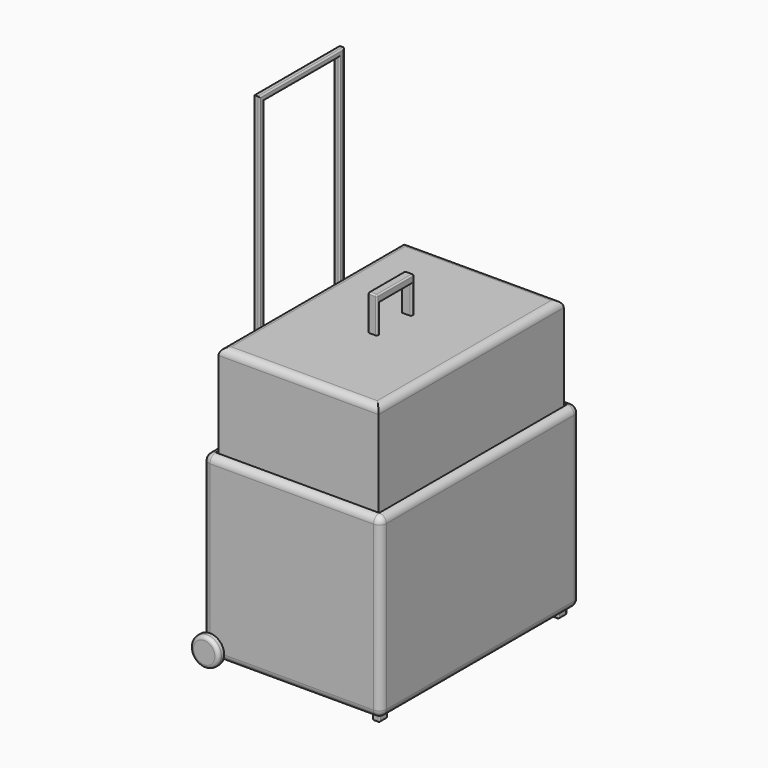
from build123d import *

# Parameters (mm, degrees)
F0_W          = 63.5
F0_H          = 88.9
F1_DEPTH      = 63.5
F2_R          = 2.54
F3_T          = 2.54
F5_W          = 57.1864917874
F5_H          = 82.6394334435
F6_DEPTH      = 63.5
F8_W          = 2.0037387299
F8_H          = 38.1
F9_DEPTH      = 127
F10_W         = 33.6400913075
F10_H         = 121.5383969247
F11_DEPTH     = 25.4
F12_R         = 2.54
F14_R         = 5.08
F15_DEPTH     = 2.54
F17_R         = 5.08
F18_DEPTH     = 2.54
F19_R         = 1.27
F20_R         = 1.27
F21_W         = 2.54
F21_H         = 3.81
F22_DEPTH     = 2.54
F23_T1_DEPTH  = 1.524
F23_T3_DEPTH  = 2.794
F23_T5_DEPTH  = 2.032
F23_S9_W      = 0.51816
F23_S9_H      = 0.51816
F23_T10_DEPTH = 0.51816
F23_S15_W     = 0.51816
F23_S15_H     = 0.51816
F23_T16_DEPTH = 0.51816
F23_S21_W     = 0.51816
F23_S21_H     = 0.51816
F23_T22_DEPTH = 0.51816
F23_S27_W     = 0.51816
F23_S27_H     = 0.51816
F23_T28_DEPTH = 0.51816
F23_T34_DEPTH = 3.302
F23_S35_R     = 2.54
F23_T36_DEPTH = 3
F23_S37_R     = 2.54
F23_T38_DEPTH = 3
F24_W         = 2.54
F24_H         = 3.81
F25_DEPTH     = 2.54
F26_T1_DEPTH  = 2.032
F26_T3_DEPTH  = 1.524
F26_T5_DEPTH  = 2.794
F26_S9_W      = 0.51816
F26_S9_H      = 0.51816
F26_T10_DEPTH = 0.51816
F26_S15_W     = 0.51816
F26_S15_H     = 0.51816
F26_T16_DEPTH = 0.51816
F26_S21_W     = 0.51816
F26_S21_H     = 0.51816
F26_T22_DEPTH = 0.51816
F26_S27_W     = 0.51816
F26_S27_H     = 0.51816
F26_T28_DEPTH = 0.51816
F26_T34_DEPTH = 3.302
F26_S35_R     = 2.54
F26_T36_DEPTH = 3
F26_S37_R     = 2.54
F26_T38_DEPTH = 3
F27_W         = 3.1932555193
F27_H         = 16.5994334435
F28_DEPTH     = 12.7
F29_W         = 14.0208706725
F29_H         = 9.9744812679
F30_DEPTH     = 25.4
F31_R         = 0.508
F32_R         = 0.508
F33_R         = 2.53999
F34_R         = 0.508


# Not quite as in the source:
# - a fillet or chamfer that OpenCascade refuses, or shapes differently, is made with other operations: its cross-section is extruded or revolved along the edge and cut away or added
# - a fillet or chamfer is up to 0.001 mm smaller than in the source, because OpenCascade refuses the exact size
# - a shell that OpenCascade refuses in one call is made with other operations: the cavity is built on its own and cut out


with BuildPart() as f1:
    # F0 (on Top) → F1 (new body)
    with BuildSketch(Plane.XY):
        with Locations((-4.3823961169, -4.1256137789)):
            Rectangle(F0_W, F0_H)
    extrude(amount=F1_DEPTH)

    # F2
    f2_edges = [f1.edges().sort_by_distance(p)[0] for p in [
        (-36.132396, -48.575614, 31.75),
        (27.367604, -48.575614, 31.75),
        (27.367604, 40.324386, 31.75),
        (27.367604, -4.125614, 0),
        (-4.382396, -48.575614, 0),
        (-4.382396, 40.324386, 0),
        (-36.132396, -4.125614, 0),
        (-36.132396, 40.324386, 31.75),
    ]]
    fillet(f2_edges, radius=F2_R)

    # F3: shell of thickness 2.54, made by hand


with BuildPart() as f3_core1:
    # F3_t2: copy of F1
    add(f1.part)

    # the walls: a layer under each face that stays
    f3_faces = [f3_core1.faces().sort_by_distance(p)[0] for p in [
        (-4.3823961169, 40.3243862211, 33.02),
        (27.3676038831, -4.1256137789, 33.02),
        (-36.1323961169, -4.1256137789, 33.02),
        (-4.3823961169, -48.5756137789, 33.02),
        (-4.3823961169, -4.1256137789, 0),
    ]]
    thicken(f3_faces, amount=-F3_T, mode=Mode.SUBTRACT)


with BuildPart() as f1_1:
    add(f1.part)

    # what is left inside the walls is the cavity
    f3_cavity = [f3_core1.part.solids().sort_by_distance(p)[0] for p in [
        (24.802204, -4.125614, 43.18),
    ]]
    add(f3_cavity, mode=Mode.SUBTRACT)

    # F14 (on offset) → F15 (join)
    with BuildSketch(Plane.XZ.offset(51.1156137789)):
        with Locations((-33.6265787482, 2.6266253553)):
            Circle(F14_R)
    extrude(amount=-F15_DEPTH)

    # F19
    f19_edges = [f1_1.edges().sort_by_distance(p)[0] for p in [
        (-38.706579, -51.115614, 2.626625),
    ]]
    fillet(f19_edges, radius=F19_R)

    # F21 (on face) → F22 (join)
    with BuildSketch(Plane(origin=(0, 0, 0), x_dir=(1, 0, 0), z_dir=(0, 0, -1))):
        with Locations((23.5576038831, 44.1306137789)):
            Rectangle(F21_W, F21_H)
    extrude(amount=F22_DEPTH)

    # F23: fillet of radius 0.508 on 8 edges, made by hand

    # F23_s2 → F23_t1 (cut)
    with BuildSketch(Plane.YZ.offset(22.7956038831)):
        with BuildLine():
            ThreePointArc((-42.2256137789, -2.032), (-42.3744035341, -2.3912102448), (-42.7336137789, -2.54))
            Line((-42.7336137789, -2.54), (-42.2256137789, -2.54))
            Line((-42.2256137789, -2.54), (-42.2256137789, -2.032))
        make_face()
        with BuildLine():
            ThreePointArc((-46.0356137789, -2.032), (-45.8868240238, -2.3912102448), (-45.5276137789, -2.54))
            Line((-45.5276137789, -2.54), (-46.0356137789, -2.54))
            Line((-46.0356137789, -2.54), (-46.0356137789, -2.032))
        make_face()
    extrude(amount=F23_T1_DEPTH, mode=Mode.SUBTRACT)

    # F23_s4 → F23_t3 (cut)
    with BuildSketch(Plane.XZ.offset(42.7336137789)):
        with BuildLine():
            ThreePointArc((22.2876038831, -2.032), (22.4363936383, -2.3912102448), (22.7956038831, -2.54))
            Line((22.7956038831, -2.54), (22.2876038831, -2.54))
            Line((22.2876038831, -2.54), (22.2876038831, -2.032))
        make_face()
        with BuildLine():
            ThreePointArc((24.8276038831, -2.032), (24.678814128, -2.3912102448), (24.3196038831, -2.54))
            Line((24.3196038831, -2.54), (24.8276038831, -2.54))
            Line((24.8276038831, -2.54), (24.8276038831, -2.032))
        make_face()
    extrude(amount=F23_T3_DEPTH, mode=Mode.SUBTRACT)

    # F23_s6 → F23_t5 (cut)
    with BuildSketch(Plane.XY.offset(-2.032)):
        with BuildLine():
            ThreePointArc((24.3196038831, -42.2256137789), (24.678814128, -42.3744035341), (24.8276038831, -42.7336137789))
            Line((24.8276038831, -42.7336137789), (24.8276038831, -42.2256137789))
            Line((24.8276038831, -42.2256137789), (24.3196038831, -42.2256137789))
        make_face()
        with BuildLine():
            ThreePointArc((22.7956038831, -42.2256137789), (22.4363936383, -42.3744035341), (22.2876038831, -42.7336137789))
            Line((22.2876038831, -42.7336137789), (22.2876038831, -42.2256137789))
            Line((22.2876038831, -42.2256137789), (22.7956038831, -42.2256137789))
        make_face()
        with BuildLine():
            ThreePointArc((22.7956038831, -46.0356137789), (22.4363936383, -45.8868240238), (22.2876038831, -45.5276137789))
            Line((22.2876038831, -45.5276137789), (22.2876038831, -46.0356137789))
            Line((22.2876038831, -46.0356137789), (22.7956038831, -46.0356137789))
        make_face()
    extrude(amount=F23_T5_DEPTH, mode=Mode.SUBTRACT)


with BuildPart() as f6:
    # F5 (on offset) → F6 (new body)
    with BuildSketch(Plane.XY.offset(33.02)):
        with Locations((-4.3823942542, -4.2082518339)):
            Rectangle(F5_W, F5_H)
    extrude(amount=F6_DEPTH)

    # F12
    f12_edges = [f6.edges().sort_by_distance(p)[0] for p in [
        (24.210852, -4.208252, 96.52),
        (-4.382394, -45.527969, 96.52),
        (-32.97564, -4.208252, 96.52),
        (-4.382394, 37.111465, 96.52),
    ]]
    fillet(f12_edges, radius=F12_R)

    # F27 (on face) → F28 (join)
    with BuildSketch(Plane.XY.offset(96.52)):
        with Locations((-4.4340703171, -4.2082518339)):
            Rectangle(F27_W, F27_H)
    extrude(amount=F28_DEPTH)

    # F29 (on face) → F30 (cut)
    with BuildSketch(Plane.YZ.offset(-2.8374425574)):
        with Locations((-4.2202234035, 101.507240634)):
            Rectangle(F29_W, F29_H)
    extrude(amount=-F30_DEPTH, mode=Mode.SUBTRACT)

    # F34
    f34_edges = [f6.edges().sort_by_distance(p)[0] for p in [
        (-2.837443, -4.208252, 109.22),
        (-2.837443, -4.220223, 106.494481),
        (-2.837443, -11.230659, 101.507241),
        (-2.837443, -12.507969, 102.87),
        (-2.837443, 2.790212, 101.507241),
        (-2.837443, 4.091465, 102.87),
        (-4.43407, -12.507969, 109.22),
        (-4.43407, 4.091465, 109.22),
        (-6.030698, -4.208252, 109.22),
        (-6.030698, -12.507969, 102.87),
        (-6.030698, 4.091465, 102.87),
        (-6.030698, -4.220223, 106.494481),
    ]]
    fillet(f34_edges, radius=F34_R)


with BuildPart() as f9:
    # F8 (on offset) → F9 (new body)
    with BuildSketch(Plane(origin=(0, 0, 38.1), x_dir=(1, 0, 0), z_dir=(0, 0, -1))):
        with Locations((-37.3555310071, 4.1256137789)):
            Rectangle(F8_W, F8_H)
    extrude(amount=-F9_DEPTH)

    # F10 (on face) → F11 (cut)
    with BuildSketch(Plane(origin=(-38.357400372, 0, 0), x_dir=(0, -1, 0), z_dir=(-1, 0, 0))):
        with Locations((4.1087935679, 102.21859999)):
            Rectangle(F10_W, F10_H)
    extrude(amount=-F11_DEPTH, mode=Mode.SUBTRACT)

    # F31
    f31_edges = [f9.edges().sort_by_distance(p)[0] for p in [
        (-36.353662, -23.175614, 101.6),
        (-36.353662, -4.125614, 165.1),
        (-36.353662, 14.924386, 101.6),
        (-36.353662, 12.711252, 102.2186),
        (-36.353662, -20.928839, 102.2186),
        (-36.353662, -4.108794, 162.987798),
    ]]
    fillet(f31_edges, radius=F31_R)

    # F32
    f32_edges = [f9.edges().sort_by_distance(p)[0] for p in [
        (-38.3574, -4.125614, 165.1),
        (-38.3574, -4.108794, 162.987798),
        (-38.3574, 12.711252, 102.2186),
        (-38.3574, -20.928839, 102.2186),
        (-38.3574, -23.175614, 101.6),
        (-38.3574, 14.924386, 101.6),
    ]]
    fillet(f32_edges, radius=F32_R)


with BuildPart() as f18:
    # F17 (on offset) → F18 (new body)
    with BuildSketch(Plane(origin=(0, 42.8643862211, 0), x_dir=(-1, 0, 0), z_dir=(0, 1, 0))):
        with Locations((33.544100821, 2.5477190502)):
            Circle(F17_R)
    extrude(amount=-F18_DEPTH)

    # F20
    f20_edges = [f18.edges().sort_by_distance(p)[0] for p in [
        (-28.464101, 42.864386, 2.547719),
    ]]
    fillet(f20_edges, radius=F20_R)


with BuildPart() as f23_tool8:
    # F23_s9 → F23_t10 (new body)
    with BuildSketch(Plane.YZ.offset(22.7956038831)):
        with Locations((-42.4745337789, -2.29108)):
            Rectangle(F23_S9_W, F23_S9_H)
    extrude(amount=-F23_T10_DEPTH)

    # F23_s11 → F23_t12 (revolve, cut)
    with BuildSketch(Plane(origin=(22.7956038831, -42.7336137789, -2.032), x_dir=(0, -0.7071067812, 0.7071067812), z_dir=(0, -0.7071067812, -0.7071067812))):
        with BuildLine():
            ThreePointArc((0, -0.508), (0.508, 0), (0, 0.508))
            Line((0, 0.508), (0, -0.508))
        make_face()
    revolve(axis=Axis((22.7956038831, -42.7336137789, -2.032), (-1, 0, 0)), mode=Mode.SUBTRACT)


with BuildPart() as f1_2:
    add(f1_1.part)

    # F23_t7: cut F23_tool8
    add(f23_tool8.part, mode=Mode.SUBTRACT)


with BuildPart() as f23_tool14:
    # F23_s15 → F23_t16 (new body)
    with BuildSketch(Plane.YZ.offset(24.3196038831)):
        with Locations((-42.4745337789, -2.29108)):
            Rectangle(F23_S15_W, F23_S15_H)
    extrude(amount=F23_T16_DEPTH)

    # F23_s17 → F23_t18 (revolve, cut)
    with BuildSketch(Plane(origin=(24.3196038831, -42.7336137789, -2.032), x_dir=(0, -0.7071067812, 0.7071067812), z_dir=(0, 0.7071067812, 0.7071067812))):
        with BuildLine():
            ThreePointArc((0, -0.508), (0.508, 0), (0, 0.508))
            Line((0, 0.508), (0, -0.508))
        make_face()
    revolve(axis=Axis((24.3196038831, -42.7336137789, -2.032), (1, 0, 0)), mode=Mode.SUBTRACT)


with BuildPart() as f1_3:
    add(f1_2.part)

    # F23_t13: cut F23_tool14
    add(f23_tool14.part, mode=Mode.SUBTRACT)


with BuildPart() as f23_tool20:
    # F23_s21 → F23_t22 (new body)
    with BuildSketch(Plane.YZ.offset(22.7956038831)):
        with Locations((-45.7866937789, -2.29108)):
            Rectangle(F23_S21_W, F23_S21_H)
    extrude(amount=-F23_T22_DEPTH)

    # F23_s23 → F23_t24 (revolve, cut)
    with BuildSketch(Plane(origin=(22.7956038831, -45.5276137789, -2.032), x_dir=(0, 0.7071067812, 0.7071067812), z_dir=(0, -0.7071067812, 0.7071067812))):
        with BuildLine():
            ThreePointArc((0, -0.508), (0.508, 0), (0, 0.508))
            Line((0, 0.508), (0, -0.508))
        make_face()
    revolve(axis=Axis((22.7956038831, -45.5276137789, -2.032), (-1, 0, 0)), mode=Mode.SUBTRACT)


with BuildPart() as f1_4:
    add(f1_3.part)

    # F23_t19: cut F23_tool20
    add(f23_tool20.part, mode=Mode.SUBTRACT)


with BuildPart() as f23_tool26:
    # F23_s27 → F23_t28 (new body)
    with BuildSketch(Plane.YZ.offset(24.3196038831)):
        with Locations((-45.7866937789, -2.29108)):
            Rectangle(F23_S27_W, F23_S27_H)
    extrude(amount=F23_T28_DEPTH)

    # F23_s29 → F23_t30 (revolve, cut)
    with BuildSketch(Plane(origin=(24.3196038831, -45.5276137789, -2.032), x_dir=(0, 0.7071067812, 0.7071067812), z_dir=(0, 0.7071067812, -0.7071067812))):
        with BuildLine():
            ThreePointArc((0, -0.508), (0.508, 0), (0, 0.508))
            Line((0, 0.508), (0, -0.508))
        make_face()
    revolve(axis=Axis((24.3196038831, -45.5276137789, -2.032), (1, 0, 0)), mode=Mode.SUBTRACT)


with BuildPart() as f1_5:
    add(f1_4.part)

    # F23_t25: cut F23_tool26
    add(f23_tool26.part, mode=Mode.SUBTRACT)


with BuildPart() as f23_tool32:
    # F23_s33 → F23_t34 (new body)
    with BuildSketch(Plane.XY.offset(1.27)):
        with BuildLine():
            ThreePointArc((24.3196038831, -46.0356137789), (24.678814128, -45.8868240238), (24.8276038831, -45.5276137789))
            Line((24.8276038831, -45.5276137789), (24.8276038831, -46.0356137789))
            Line((24.8276038831, -46.0356137789), (24.3196038831, -46.0356137789))
        make_face()
    extrude(amount=-F23_T34_DEPTH)

    # F23_s35 → F23_t36 (cut, symmetric)
    with BuildSketch(Plane.YZ.offset(24.6)):
        with Locations((-46.0356137789, 2.54)):
            Circle(F23_S35_R)
    extrude(amount=F23_T36_DEPTH, both=True, mode=Mode.SUBTRACT)

    # F23_s37 → F23_t38 (cut, symmetric)
    with BuildSketch(Plane.XZ.offset(45.8)):
        with Locations((24.8276038831, 2.54)):
            Circle(F23_S37_R)
    extrude(amount=F23_T38_DEPTH, both=True, mode=Mode.SUBTRACT)


with BuildPart() as f1_6:
    add(f1_5.part)

    # F23_t31: cut F23_tool32
    add(f23_tool32.part, mode=Mode.SUBTRACT)

    # F24 (on face) → F25 (join)
    with BuildSketch(Plane(origin=(0, 0, 0), x_dir=(1, 0, 0), z_dir=(0, 0, -1))):
        with Locations((23.5576038831, -35.8793862211)):
            Rectangle(F24_W, F24_H)
    extrude(amount=F25_DEPTH)

    # F26: fillet of radius 0.508 on 8 edges, made by hand

    # F26_s2 → F26_t1 (cut)
    with BuildSketch(Plane.XY.offset(-2.032)):
        with BuildLine():
            ThreePointArc((22.2876038831, 37.2763862211), (22.4363936383, 37.6355964659), (22.7956038831, 37.7843862211))
            Line((22.7956038831, 37.7843862211), (22.2876038831, 37.7843862211))
            Line((22.2876038831, 37.7843862211), (22.2876038831, 37.2763862211))
        make_face()
        with BuildLine():
            ThreePointArc((24.3196038831, 33.9743862211), (24.678814128, 34.1231759762), (24.8276038831, 34.4823862211))
            Line((24.8276038831, 34.4823862211), (24.8276038831, 33.9743862211))
            Line((24.8276038831, 33.9743862211), (24.3196038831, 33.9743862211))
        make_face()
        with BuildLine():
            ThreePointArc((22.2876038831, 34.4823862211), (22.4363936383, 34.1231759762), (22.7956038831, 33.9743862211))
            Line((22.7956038831, 33.9743862211), (22.2876038831, 33.9743862211))
            Line((22.2876038831, 33.9743862211), (22.2876038831, 34.4823862211))
        make_face()
    extrude(amount=F26_T1_DEPTH, mode=Mode.SUBTRACT)

    # F26_s4 → F26_t3 (cut)
    with BuildSketch(Plane.YZ.offset(22.7956038831)):
        with BuildLine():
            ThreePointArc((37.7843862211, -2.032), (37.6355964659, -2.3912102448), (37.2763862211, -2.54))
            Line((37.2763862211, -2.54), (37.7843862211, -2.54))
            Line((37.7843862211, -2.54), (37.7843862211, -2.032))
        make_face()
        with BuildLine():
            ThreePointArc((33.9743862211, -2.032), (34.1231759762, -2.3912102448), (34.4823862211, -2.54))
            Line((34.4823862211, -2.54), (33.9743862211, -2.54))
            Line((33.9743862211, -2.54), (33.9743862211, -2.032))
        make_face()
    extrude(amount=F26_T3_DEPTH, mode=Mode.SUBTRACT)

    # F26_s6 → F26_t5 (cut)
    with BuildSketch(Plane.XZ.offset(-37.2763862211)):
        with BuildLine():
            ThreePointArc((22.2876038831, -2.032), (22.4363936383, -2.3912102448), (22.7956038831, -2.54))
            Line((22.7956038831, -2.54), (22.2876038831, -2.54))
            Line((22.2876038831, -2.54), (22.2876038831, -2.032))
        make_face()
        with BuildLine():
            ThreePointArc((24.3196038831, -2.54), (24.678814128, -2.3912102448), (24.8276038831, -2.032))
            Line((24.8276038831, -2.032), (24.8276038831, -2.54))
            Line((24.8276038831, -2.54), (24.3196038831, -2.54))
        make_face()
    extrude(amount=F26_T5_DEPTH, mode=Mode.SUBTRACT)


with BuildPart() as f26_tool8:
    # F26_s9 → F26_t10 (new body)
    with BuildSketch(Plane.XZ.offset(-37.2763862211)):
        with Locations((24.5786838831, -2.29108)):
            Rectangle(F26_S9_W, F26_S9_H)
    extrude(amount=-F26_T10_DEPTH)

    # F26_s11 → F26_t12 (revolve, cut)
    with BuildSketch(Plane(origin=(24.3196038831, 37.2763862211, -2.032), x_dir=(-0.7071067812, 0, 0.7071067812), z_dir=(-0.7071067812, 0, -0.7071067812))):
        with BuildLine():
            ThreePointArc((0, -0.508), (0.508, 0), (0, 0.508))
            Line((0, 0.508), (0, -0.508))
        make_face()
    revolve(axis=Axis((24.3196038831, 37.2763862211, -2.032), (0, 1, 0)), mode=Mode.SUBTRACT)


with BuildPart() as f1_7:
    add(f1_6.part)

    # F26_t7: cut F26_tool8
    add(f26_tool8.part, mode=Mode.SUBTRACT)


with BuildPart() as f26_tool14:
    # F26_s15 → F26_t16 (new body)
    with BuildSketch(Plane.XZ.offset(-37.2763862211)):
        with Locations((22.5365238831, -2.29108)):
            Rectangle(F26_S15_W, F26_S15_H)
    extrude(amount=-F26_T16_DEPTH)

    # F26_s17 → F26_t18 (revolve, cut)
    with BuildSketch(Plane(origin=(22.7956038831, 37.2763862211, -2.032), x_dir=(0.7071067812, 0, 0.7071067812), z_dir=(-0.7071067812, 0, 0.7071067812))):
        with BuildLine():
            ThreePointArc((0, -0.508), (0.508, 0), (0, 0.508))
            Line((0, 0.508), (0, -0.508))
        make_face()
    revolve(axis=Axis((22.7956038831, 37.2763862211, -2.032), (0, 1, 0)), mode=Mode.SUBTRACT)


with BuildPart() as f1_8:
    add(f1_7.part)

    # F26_t13: cut F26_tool14
    add(f26_tool14.part, mode=Mode.SUBTRACT)


with BuildPart() as f26_tool20:
    # F26_s21 → F26_t22 (new body)
    with BuildSketch(Plane.XY.offset(-2.032)):
        with Locations((22.5365238831, 34.2233062211)):
            Rectangle(F26_S21_W, F26_S21_H)
    extrude(amount=-F26_T22_DEPTH)

    # F26_s23 → F26_t24 (revolve, cut)
    with BuildSketch(Plane(origin=(22.7956038831, 34.4823862211, -2.032), x_dir=(0.7071067812, 0.7071067812, 0), z_dir=(-0.7071067812, 0.7071067812, 0))):
        with BuildLine():
            ThreePointArc((0, -0.508), (0.508, 0), (0, 0.508))
            Line((0, 0.508), (0, -0.508))
        make_face()
    revolve(axis=Axis((22.7956038831, 34.4823862211, -2.032), (0, 0, -1)), mode=Mode.SUBTRACT)


with BuildPart() as f1_9:
    add(f1_8.part)

    # F26_t19: cut F26_tool20
    add(f26_tool20.part, mode=Mode.SUBTRACT)


with BuildPart() as f26_tool26:
    # F26_s27 → F26_t28 (new body)
    with BuildSketch(Plane.XY.offset(-2.032)):
        with Locations((24.5786838831, 34.2233062211)):
            Rectangle(F26_S27_W, F26_S27_H)
    extrude(amount=-F26_T28_DEPTH)

    # F26_s29 → F26_t30 (revolve, cut)
    with BuildSketch(Plane(origin=(24.3196038831, 34.4823862211, -2.032), x_dir=(-0.7071067812, 0.7071067812, 0), z_dir=(-0.7071067812, -0.7071067812, 0))):
        with BuildLine():
            ThreePointArc((0, -0.508), (0.508, 0), (0, 0.508))
            Line((0, 0.508), (0, -0.508))
        make_face()
    revolve(axis=Axis((24.3196038831, 34.4823862211, -2.032), (0, 0, -1)), mode=Mode.SUBTRACT)


with BuildPart() as f1_10:
    add(f1_9.part)

    # F26_t25: cut F26_tool26
    add(f26_tool26.part, mode=Mode.SUBTRACT)


with BuildPart() as f26_tool32:
    # F26_s33 → F26_t34 (new body)
    with BuildSketch(Plane.XY.offset(1.27)):
        with BuildLine():
            ThreePointArc((24.3196038831, 37.7843862211), (24.678814128, 37.6355964659), (24.8276038831, 37.2763862211))
            Line((24.8276038831, 37.2763862211), (24.8276038831, 37.7843862211))
            Line((24.8276038831, 37.7843862211), (24.3196038831, 37.7843862211))
        make_face()
    extrude(amount=-F26_T34_DEPTH)

    # F26_s35 → F26_t36 (cut, symmetric)
    with BuildSketch(Plane.YZ.offset(24.6)):
        with Locations((37.7843862211, 2.54)):
            Circle(F26_S35_R)
    extrude(amount=F26_T36_DEPTH, both=True, mode=Mode.SUBTRACT)

    # F26_s37 → F26_t38 (cut, symmetric)
    with BuildSketch(Plane.XZ.offset(-37.5)):
        with Locations((24.8276038831, 2.54)):
            Circle(F26_S37_R)
    extrude(amount=F26_T38_DEPTH, both=True, mode=Mode.SUBTRACT)


with BuildPart() as f1_11:
    add(f1_10.part)

    # F26_t31: cut F26_tool32
    add(f26_tool32.part, mode=Mode.SUBTRACT)

    # F33 (radius 2.54 in the source; OpenCascade refuses exactly that, so slightly less here)
    f33_edges = [f1_11.edges().sort_by_distance(p)[0] for p in [
        (27.367604, -4.125614, 63.5),
        (-4.382396, -48.575614, 63.5),
        (-4.382396, 40.324386, 63.5),
        (-36.132396, -4.125614, 63.5),
        (-35.388447, -47.831665, 63.5),
        (26.623655, -47.831665, 63.5),
        (26.623655, 39.580437, 63.5),
        (-35.388447, 39.580437, 63.5),
    ]]
    fillet(f33_edges, radius=F33_R)


solid = Compound([f6.part, f9.part, f18.part, f1_11.part])
